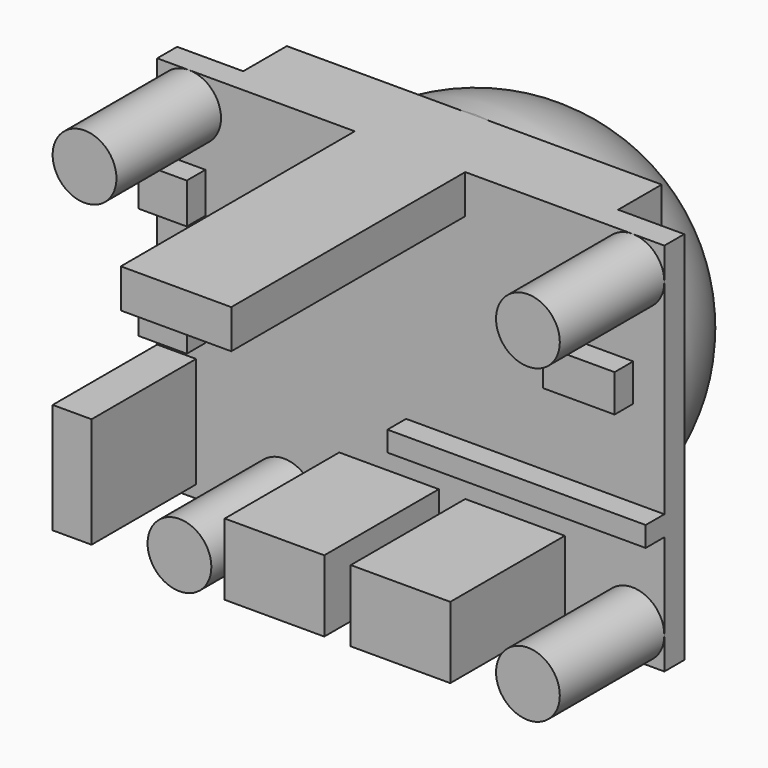
from build123d import *

# Parameters (mm, degrees)
F2_DEPTH = 1.6
F3_DEPTH = 5.1
F4_DEPTH = 17.2
F1_R     = 2.05
F1_W     = 2.5
F1_H     = 7.1
F1_W_2   = 7.1
F1_H_2   = 2.5
F6_DEPTH = 8.4
F1_W_3   = 6.4
F1_H_3   = 4.6
F7_DEPTH = 9.2
F8_DEPTH = 18.8
F1_W_4   = 3.1
F1_H_4   = 1.3
F1_W_5   = 4.6
F1_H_5   = 2.4
F1_W_6   = 16.6
F1_H_6   = 2.6
F9_DEPTH = 1.5


# Not quite as in the source:
# - a fillet or chamfer that OpenCascade refuses, or shapes differently, is made with other operations: its cross-section is extruded or revolved along the edge and cut away or added


with BuildPart() as f2:
    # F0 (on Front) → F2 (new body)
    with BuildSketch(Plane.XZ):
        Polygon((16.3, -12.05), (16.3, 12.05), (12.05, 12.05), (12.05, 0), (12.05, -12.05), align=None)
        with BuildLine():
            Line((12.05, 0), (12.05, 12.05))
            Line((12.05, 12.05), (0, 12.05))
            ThreePointArc((0, 12.05), (8.5206367133, 8.5206367133), (12.05, 0))
        make_face()
        with BuildLine():
            ThreePointArc((-12.05, 0), (-8.5206367133, 8.5206367133), (0, 12.05))
            Line((0, 12.05), (-12.05, 12.05))
            Line((-12.05, 12.05), (-12.05, 0))
        make_face()
        with BuildLine():
            ThreePointArc((12.05, 0), (8.5206367133, 8.5206367133), (0, 12.05))
            ThreePointArc((0, 12.05), (-8.5206367133, 8.5206367133), (-12.05, 0))
            ThreePointArc((-12.05, 0), (-8.5206367125, -8.5206367141), (2.1e-09, -12.05))
            ThreePointArc((2.1e-09, -12.05), (8.5206367141, -8.5206367125), (12.05, 0))
        make_face()
        with BuildLine():
            Line((12.05, -12.05), (12.05, 0))
            ThreePointArc((12.05, 0), (8.5206367141, -8.5206367125), (2.1e-09, -12.05))
            Line((2.1e-09, -12.05), (12.05, -12.05))
        make_face()
        Polygon((-12.05, 0), (-12.05, 12.05), (-16.3, 12.05), (-16.3, -12.05), (-12.05, -12.05), align=None)
        with BuildLine():
            ThreePointArc((2.1e-09, -12.05), (-8.5206367125, -8.5206367141), (-12.05, 0))
            Line((-12.05, 0), (-12.05, -12.05))
            Line((-12.05, -12.05), (2.1e-09, -12.05))
        make_face()
    extrude(amount=-F2_DEPTH)

    # F0 (on Front) → F3 (join)
    with BuildSketch(Plane.XZ):
        with BuildLine():
            ThreePointArc((2.1e-09, -12.05), (-8.5206367125, -8.5206367141), (-12.05, 0))
            Line((-12.05, 0), (-12.05, -12.05))
            Line((-12.05, -12.05), (2.1e-09, -12.05))
        make_face()
        with BuildLine():
            ThreePointArc((-12.05, 0), (-8.5206367133, 8.5206367133), (0, 12.05))
            Line((0, 12.05), (-12.05, 12.05))
            Line((-12.05, 12.05), (-12.05, 0))
        make_face()
        with BuildLine():
            ThreePointArc((12.05, 0), (8.5206367133, 8.5206367133), (0, 12.05))
            ThreePointArc((0, 12.05), (-8.5206367133, 8.5206367133), (-12.05, 0))
            ThreePointArc((-12.05, 0), (-8.5206367125, -8.5206367141), (2.1e-09, -12.05))
            ThreePointArc((2.1e-09, -12.05), (8.5206367141, -8.5206367125), (12.05, 0))
        make_face()
        with BuildLine():
            Line((12.05, 0), (12.05, 12.05))
            Line((12.05, 12.05), (0, 12.05))
            ThreePointArc((0, 12.05), (8.5206367133, 8.5206367133), (12.05, 0))
        make_face()
        with BuildLine():
            Line((12.05, -12.05), (12.05, 0))
            ThreePointArc((12.05, 0), (8.5206367141, -8.5206367125), (2.1e-09, -12.05))
            Line((2.1e-09, -12.05), (12.05, -12.05))
        make_face()
    extrude(amount=-F3_DEPTH)

    # F0 (on Front) → F4 (join)
    with BuildSketch(Plane.XZ):
        with BuildLine():
            ThreePointArc((12.05, 0), (8.5206367133, 8.5206367133), (0, 12.05))
            ThreePointArc((0, 12.05), (-8.5206367133, 8.5206367133), (-12.05, 0))
            ThreePointArc((-12.05, 0), (-8.5206367125, -8.5206367141), (2.1e-09, -12.05))
            ThreePointArc((2.1e-09, -12.05), (8.5206367141, -8.5206367125), (12.05, 0))
        make_face()
    extrude(amount=-F4_DEPTH)

    # F5: fillet of radius 12 on 1 edges, made by hand

    # F5_s1 → F5_t2 (revolve, cut)
    with BuildSketch(Plane.YZ):
        with BuildLine():
            ThreePointArc((5.2, -12.05), (13.6852813742, -8.5352813742), (17.2, -0.05))
            Line((17.2, -0.05), (17.2, -12.05))
            Line((17.2, -12.05), (5.2, -12.05))
        make_face()
    revolve(axis=Axis((0, 17.2, 0), (0, -1, 0)), mode=Mode.SUBTRACT)

    # F1 (on Front) → F6 (join)
    with BuildSketch(Plane.XZ):
        with Locations((-14.25, 10)):
            Circle(F1_R)
        with Locations((14.25, 10)):
            Circle(F1_R)
        with Locations((14.25, -10)):
            Circle(F1_R)
        with Locations((-8.15, -10)):
            Circle(F1_R)
        with Locations((-15.05, -7.7)):
            Rectangle(F1_W, F1_H)
        with Locations((-0.05, 10.8)):
            Rectangle(F1_W_2, F1_H_2)
    extrude(amount=F6_DEPTH)

    # F1 (on Front) → F7 (join)
    with BuildSketch(Plane.XZ):
        with Locations((-1.4, -8.75)):
            Rectangle(F1_W_3, F1_H_3)
        with Locations((6.7, -8.75)):
            Rectangle(F1_W_3, F1_H_3)
    extrude(amount=F7_DEPTH)

    # F1 (on Front) → F8 (join)
    with BuildSketch(Plane.XZ):
        with Locations((-0.05, 10.8)):
            Rectangle(F1_W_2, F1_H_2)
    extrude(amount=F8_DEPTH)

    # F1 (on Front) → F9 (join)
    with BuildSketch(Plane.XZ):
        with Locations((-14.75, -2.4)):
            Rectangle(F1_W_4, F1_H_4)
        with Locations((12, 3.65)):
            Rectangle(F1_W_5, F1_H_5)
        with Locations((8, -3.8)):
            Rectangle(F1_W_6, F1_H_4)
        with Locations((-14.75, 5.45)):
            Rectangle(F1_W_4, F1_H_6)
    extrude(amount=F9_DEPTH)


solid = f2.part
